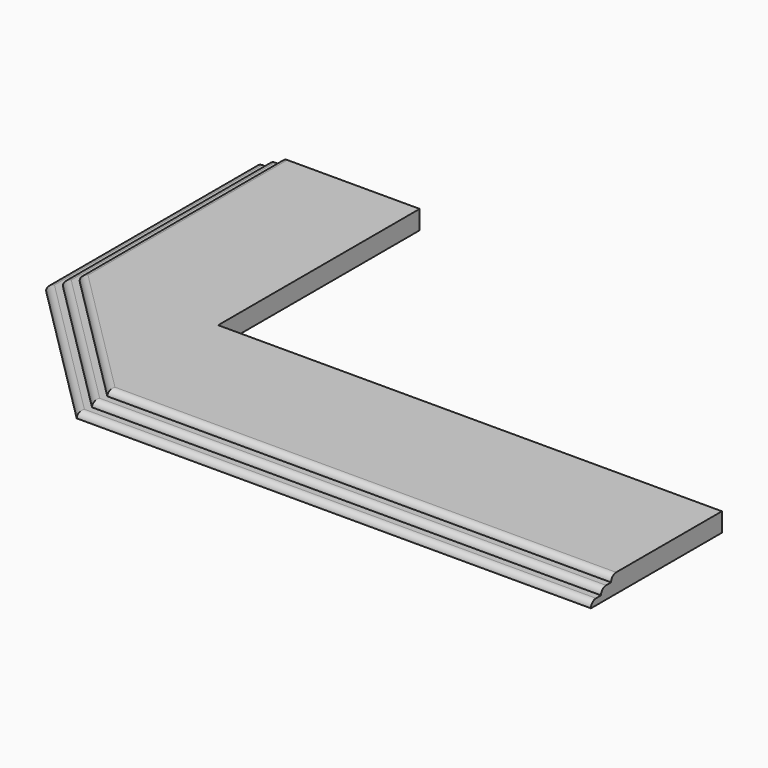
from build123d import *

# Parameters (mm, degrees)
F1_DEPTH = 25
F3_DEPTH = 25
F5_DEPTH = 25
F7_DEPTH = 720
F8_R     = 24.99999


# Not quite as in the source:
# - a fillet or chamfer is up to 0.001 mm smaller than in the source, because OpenCascade refuses the exact size


with BuildPart() as f1:
    # F0 (on Top) → F1 (new body)
    with BuildSketch(Plane.XY):
        Polygon((-1000, -500), (-1000, 500), (-1550, 500), (-1550, -500), (-1000, -1050), (1000, -1050), (1000, -500), align=None)
    extrude(amount=F1_DEPTH)

    # F2 (on face) → F3 (join)
    with BuildSketch(Plane(origin=(0, 0, 0), x_dir=(1, 0, 0), z_dir=(0, 0, -1))):
        Polygon((-1020.7106781187, 1100), (-1600, 520.7106781187), (-1600, -550), (-950, -550), (-950, 450), (1050, 450), (1050, 1100), align=None)
    extrude(amount=F3_DEPTH)

    # F4 (on face) → F5 (join)
    with BuildSketch(Plane(origin=(0, 0, -25), x_dir=(1, 0, 0), z_dir=(0, 0, -1))):
        Polygon((-1041.4213562373, 1150), (-1650, 541.4213562373), (-1650, -600), (-900, -600), (-900, 400), (1100, 400), (1100, 1150), align=None)
    extrude(amount=F5_DEPTH)

    # F6 (on face) → F7 (cut)
    with BuildSketch(Plane.XY.offset(25)):
        Polygon((-1950.9481191635, 705.582857132), (-1946.2337493896, 500), (-1000, 500), (-1000, -500), (1000, -500), (1000, -1340.4409885406), (1594.2358970642, -1340.4409885406), (1594.2358970642, 705.582857132), align=None)
    extrude(amount=-F7_DEPTH, mode=Mode.SUBTRACT)

    # F8 (radius 25 in the source; OpenCascade refuses exactly that, so slightly less here)
    f8_edges = [f1.edges().sort_by_distance(p)[0] for p in [
        (-1550, 0, 25),
        (-1600, -10.355339, 0),
        (-1650, -20.710678, -25),
        (-1275, -775, 25),
        (-1310.355339, -810.355339, 0),
        (-1345.710678, -845.710678, -25),
        (0, -1050, 25),
        (-10.355339, -1100, 0),
        (-20.710678, -1150, -25),
    ]]
    fillet(f8_edges, radius=F8_R)


solid = f1.part
